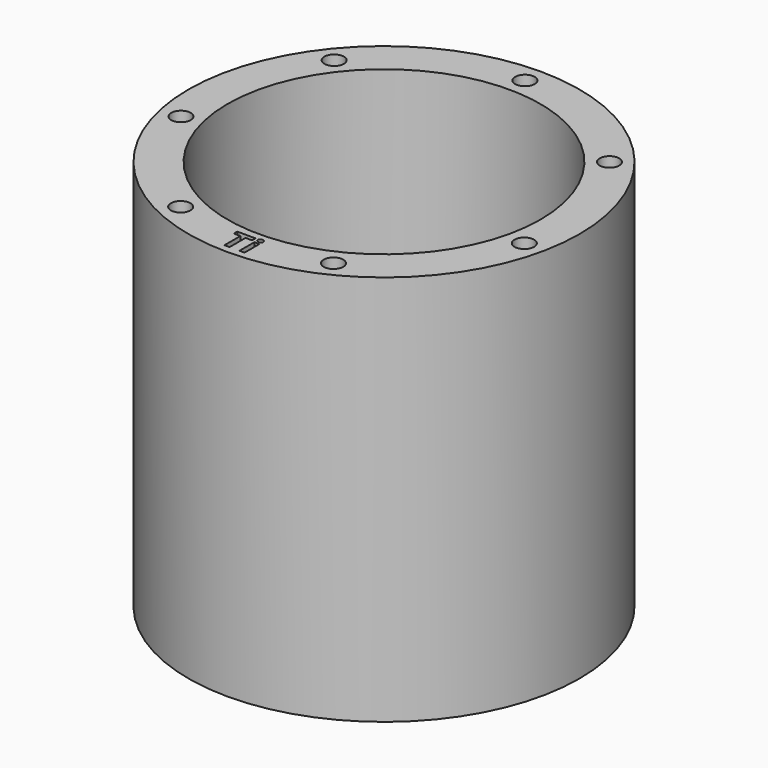
from build123d import *

# Parameters (mm, degrees)
F0_R         = 20
F0_R_2       = 1
F0_R_3       = 16
F1_DEPTH     = 40
F2_TEXT_SIZE = 3.4696448387
F3_DEPTH     = 2


# Not quite as in the source:
# - Text() gives the source's letters only with a copy of the font that has no kerning and outlines rounded to 1/6400 em; it was checked with that copy


with BuildPart() as f1:
    # F0 (on Top) → F1 (new body)
    with BuildSketch(Plane.XY):
        Circle(F0_R)
        with Locations((-7.8099073041, -16.2174396222)):
            Circle(F0_R_2, mode=Mode.SUBTRACT)
        with Locations((-17.5487024193, -4.0053768112)):
            Circle(F0_R_2, mode=Mode.SUBTRACT)
        with Locations((7.8099073041, -16.2174396222)):
            Circle(F0_R_2, mode=Mode.SUBTRACT)
        with Locations((17.5487024193, -4.0053768112)):
            Circle(F0_R_2, mode=Mode.SUBTRACT)
        with Locations((-14.0729666844, 11.2228164335)):
            Circle(F0_R_2, mode=Mode.SUBTRACT)
        Circle(F0_R_3, mode=Mode.SUBTRACT)
        with Locations((0, 18)):
            Circle(F0_R_2, mode=Mode.SUBTRACT)
        with Locations((14.0729666844, 11.2228164335)):
            Circle(F0_R_2, mode=Mode.SUBTRACT)
    extrude(amount=F1_DEPTH)

    # F2 (on face) → F3 (cut)
    with BuildSketch(Plane.XY.offset(40)):
        with Locations((-1.6764267348, -19.219731912)):
            Text('Ti', F2_TEXT_SIZE, font='Open Sans', font_style=FontStyle.BOLD, text_align=(TextAlign.LEFT, TextAlign.BOTTOM))
    extrude(amount=-F3_DEPTH, mode=Mode.SUBTRACT)


solid = f1.part
